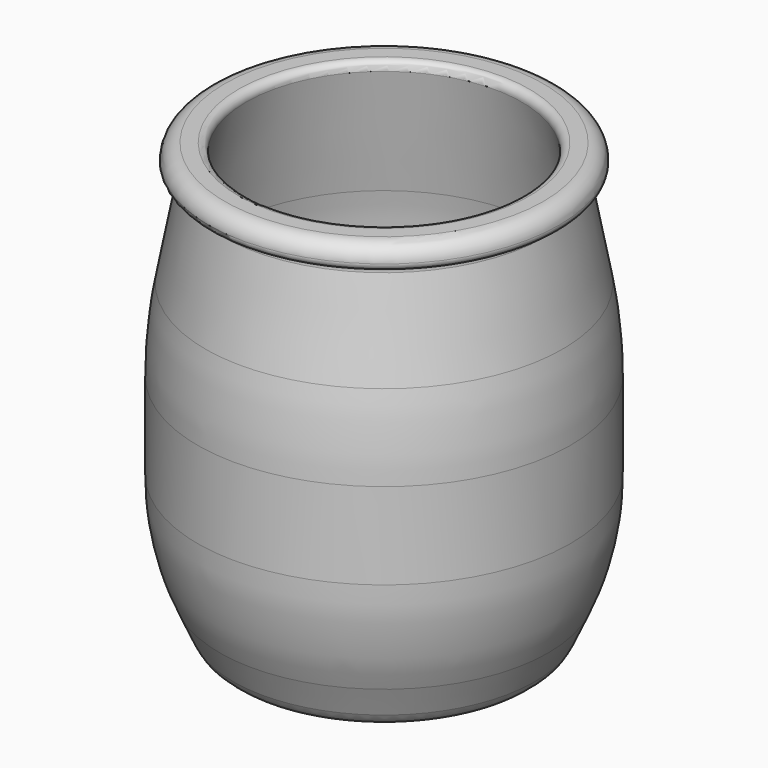
from build123d import *

# Parameters (mm, degrees)
F2_R = 2.5
F3_R = 1.19999
F4_R = 1
F5_R = 70
F6_R = 40
F7_R = 4


# Not quite as in the source:
# - a fillet or chamfer is up to 0.001 mm smaller than in the source, because OpenCascade refuses the exact size


with BuildPart() as f1:
    # F0 (on Front) → F1 (revolve)
    with BuildSketch(Plane.XZ):
        Polygon((-21.5944710413, 70), (-27.8, 70), (-27.8, 66.3), (-25.35, 66.3), (-29.6, 43.9), (-29.6, 15), (-22.85, 0), (0, 1), (0, 4.0028715148), (-20.9489735102, 3.0860674224), (-26.6, 15.6439040665), (-26.6, 43.6179179589), align=None)
    revolve(axis=Axis((0, 0, 35.5), (0, 0, -1)))

    # F2
    f2_edges = [f1.edges().sort_by_distance(p)[0] for p in [
        (27.8, 0, 70),
    ]]
    fillet(f2_edges, radius=F2_R)

    # F3 (radius 1.2 in the source; OpenCascade refuses exactly that, so slightly less here)
    f3_edges = [f1.edges().sort_by_distance(p)[0] for p in [
        (27.8, 0, 66.3),
        (21.594471, 0, 70),
    ]]
    fillet(f3_edges, radius=F3_R)

    # F4
    f4_edges = [f1.edges().sort_by_distance(p)[0] for p in [
        (25.35, 0, 66.3),
    ]]
    fillet(f4_edges, radius=F4_R)

    # F5
    f5_edges = [f1.edges().sort_by_distance(p)[0] for p in [
        (29.6, 0, 43.9),
        (26.6, 0, 43.617918),
    ]]
    fillet(f5_edges, radius=F5_R)

    # F6
    f6_edges = [f1.edges().sort_by_distance(p)[0] for p in [
        (29.6, 0, 15),
        (26.6, 0, 15.643904),
    ]]
    fillet(f6_edges, radius=F6_R)

    # F7
    f7_edges = [f1.edges().sort_by_distance(p)[0] for p in [
        (20.948974, 0, 3.086067),
        (22.85, 0, 0),
    ]]
    fillet(f7_edges, radius=F7_R)


solid = f1.part
